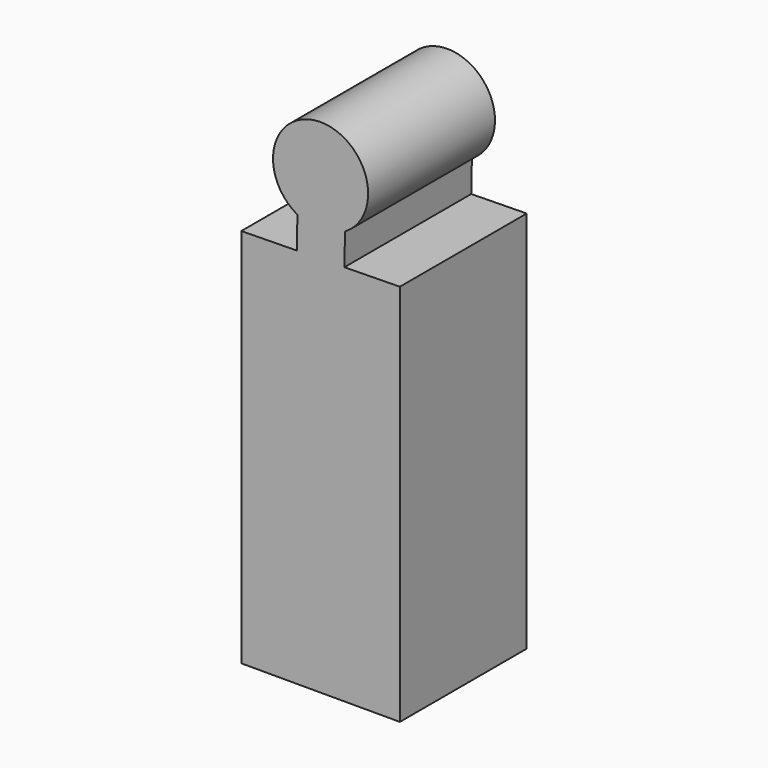
from build123d import *

# Parameters (mm, degrees)
F1_DEPTH = 50


# Not quite as in the source:
# - a feature names something its author has since deleted; it is built from what else it names


with BuildPart() as f1:
    # F0 (on Front) → F1 (new body)
    with BuildSketch(Plane.XZ):
        with BuildLine():
            Line((0, 0), (0, -120))
            Line((0, -120), (50, -120))
            Line((50, -120), (50, 0.8005096136))
            Line((50, 0.8005096136), (32.5041198008, 0.5203972077))
            Line((32.5041198008, 0.5203972077), (32.7120246633, 10.5182357525))
            ThreePointArc((32.7120246633, 10.5182357525), (25.2401221113, 8.3857971686), (17.7037850617, 10.2779509508))
            Line((17.7037850617, 10.2779509508), (17.4958801992, 0.280112406))
            Line((17.4958801992, 0.280112406), (0, 0))
        make_face()
        with BuildLine():
            ThreePointArc((40, 23.3838750912), (17.3987903619, 36.3152946589), (17.7037850617, 10.2779509508))
            ThreePointArc((17.7037850617, 10.2779509508), (25.2401221113, 8.3857971686), (32.7120246633, 10.5182357525))
            ThreePointArc((32.7120246633, 10.5182357525), (38.0514437889, 15.9906474452), (40, 23.3838750912))
        make_face()
    extrude(amount=F1_DEPTH)


solid = f1.part
